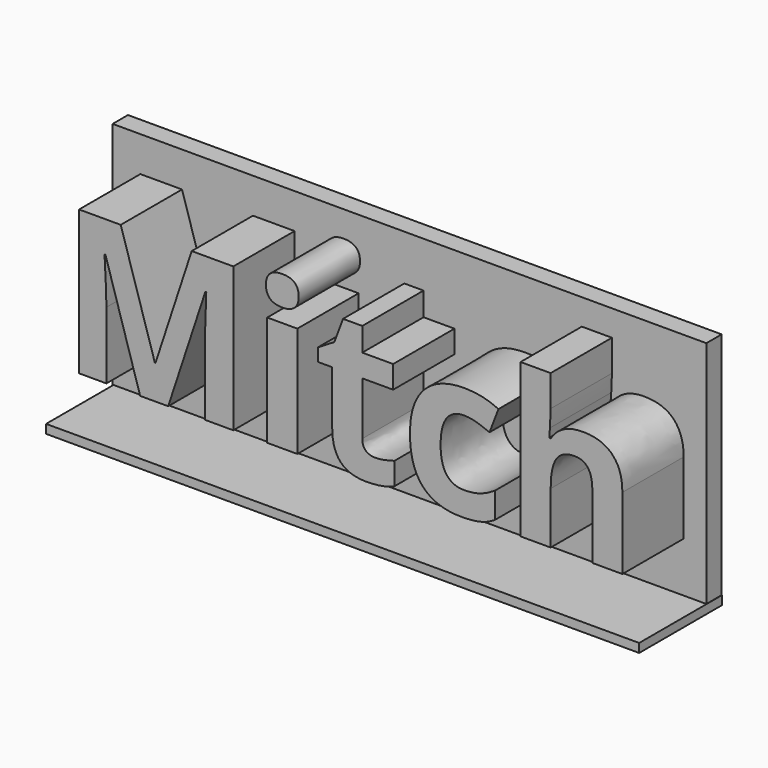
from build123d import *

# Parameters (mm, degrees)
F0_TEXT_SIZE = 52.7588480985
F1_DEPTH     = 25
F2_W         = 155
F2_H         = 60
F3_DEPTH     = 5
F4_W         = 154.8394933343
F4_H         = 2.3024464026
F5_DEPTH     = 27


# Not quite as in the source:
# - Text() gives the source's letters only with a copy of the font that has no kerning and outlines rounded to 1/6400 em; it was checked with that copy


with BuildPart() as f1:
    # F0 (on Front) → F1 (new body)
    with BuildSketch(Plane.XZ):
        with Locations((-75, 30.4936471419)):
            Text('Mitch', F0_TEXT_SIZE, font='Open Sans', font_style=FontStyle.BOLD, text_align=(TextAlign.LEFT, TextAlign.BOTTOM))
    extrude(amount=F1_DEPTH)

    # F2 (on Front) → F3 (join)
    with BuildSketch(Plane.XZ):
        with Locations((0, 47.3440466449)):
            Rectangle(F2_W, F2_H)
    extrude(amount=F3_DEPTH)

    # F4 (on Front) → F5 (join)
    with BuildSketch(Plane.XZ):
        with Locations((0.1439042389, 16.2610257976)):
            Rectangle(F4_W, F4_H)
    extrude(amount=F5_DEPTH)


solid = f1.part
